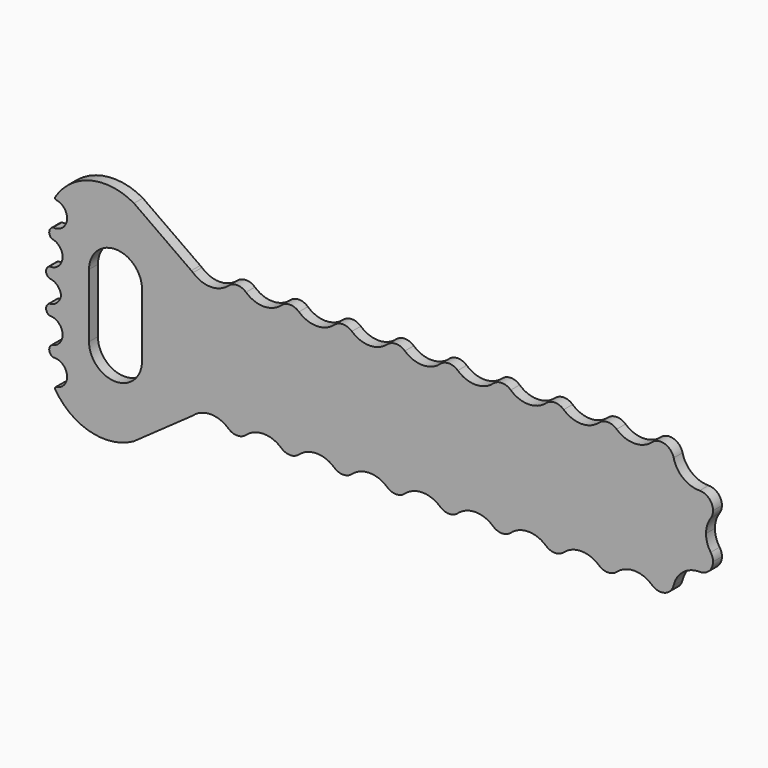
from build123d import *

# Parameters (mm, degrees)
F0_TEXT_SIZE = 24.3191204023
F1_DEPTH     = 2.667


# Not quite as in the source:
# - Text() gives the source's letters only with a copy of the font that has no kerning and outlines rounded to 1/6400 em; it was checked with that copy


with BuildPart() as f1:
    # F0 (on Front) → F1 (new body)
    with BuildSketch(Plane.XZ):
        with BuildLine():
            ThreePointArc((-63.1726785847, 1.1586809485), (-62.3909800512, 0.0883639945), (-62.1143452513, -1.2078243277))
            ThreePointArc((-62.1143452513, -1.2078243277), (-68.0745680167, -2.732015637), (-63.5777525882, 1.4663251737))
            Line((-63.5777525882, 1.4663251737), (-77.3401691147, 11.2148536242))
            ThreePointArc((-77.3401691147, 11.2148536242), (-87.8068892458, 12.6196854607), (-96.2739288474, 6.3081861795))
            ThreePointArc((-96.2739288474, 6.3081861795), (-96.2289020352, 6.0064040212), (-95.9839214808, 5.8245128095))
            ThreePointArc((-95.9839214808, 5.8245128095), (-93.4015593805, 2.4408889862), (-96.7397936857, -0.199886642))
            ThreePointArc((-96.7397936857, -0.199886642), (-97.6524269014, -1.3446739458), (-97.0623695413, -2.6845506823))
            ThreePointArc((-97.0623695413, -2.6845506823), (-94.4816228819, -5.9852371965), (-97.6549069574, -8.7211196796))
            ThreePointArc((-97.6549069574, -8.7211196796), (-98.4182841729, -9.9748064549), (-97.6549069574, -11.2284932301))
            ThreePointArc((-97.6549069574, -11.2284932301), (-95.7570755771, -12.0560699309), (-94.8309801189, -13.9078243277))
            ThreePointArc((-94.8309801189, -13.9078243277), (-95.7570755771, -15.7595787244), (-97.6549069574, -16.5871554253))
            ThreePointArc((-97.6549069574, -16.5871554253), (-98.4182841729, -17.8408422005), (-97.6549069574, -19.0945289757))
            ThreePointArc((-97.6549069574, -19.0945289757), (-94.4816228819, -21.8304114589), (-97.0623695413, -25.131097973))
            ThreePointArc((-97.0623695413, -25.131097973), (-97.6524269014, -26.4709747096), (-96.7397936857, -27.6157620133))
            ThreePointArc((-96.7397936857, -27.6157620133), (-93.4015593805, -30.2565376416), (-95.9839214808, -33.6401614649))
            ThreePointArc((-95.9839214808, -33.6401614649), (-96.2289020352, -33.8220526766), (-96.2739288474, -34.1238348349))
            ThreePointArc((-96.2739288474, -34.1238348349), (-87.8068892458, -40.4353341161), (-77.3401691147, -39.0305022795))
            Line((-77.3401691147, -39.0305022795), (-63.5777525882, -29.281973829))
            ThreePointArc((-63.5777525882, -29.281973829), (-68.0745680167, -25.0836330184), (-62.1143452513, -26.6078243277))
            ThreePointArc((-62.1143452513, -26.6078243277), (-62.3909800512, -27.9040126499), (-63.1726785847, -28.9743296039))
            ThreePointArc((-63.1726785847, -28.9743296039), (-58.9393452513, -27.3573401562), (-54.706011918, -28.9743296039))
            ThreePointArc((-54.706011918, -28.9743296039), (-53.8855335735, -23.7094591276), (-49.4143452513, -26.6078243277))
            ThreePointArc((-49.4143452513, -26.6078243277), (-49.6909800512, -27.9040126499), (-50.4726785847, -28.9743296039))
            ThreePointArc((-50.4726785847, -28.9743296039), (-46.2393452513, -27.3573401562), (-42.006011918, -28.9743296039))
            ThreePointArc((-42.006011918, -28.9743296039), (-41.1855335735, -23.7094591276), (-36.7143452513, -26.6078243277))
            ThreePointArc((-36.7143452513, -26.6078243277), (-36.9909800512, -27.9040126499), (-37.7726785847, -28.9743296039))
            ThreePointArc((-37.7726785847, -28.9743296039), (-33.5393452513, -27.3573401562), (-29.306011918, -28.9743296039))
            ThreePointArc((-29.306011918, -28.9743296039), (-28.4855335735, -23.7094591276), (-24.0143452513, -26.6078243277))
            ThreePointArc((-24.0143452513, -26.6078243277), (-24.2909800512, -27.9040126499), (-25.0726785847, -28.9743296039))
            ThreePointArc((-25.0726785847, -28.9743296039), (-20.8393452513, -27.3573401562), (-16.606011918, -28.9743296039))
            ThreePointArc((-16.606011918, -28.9743296039), (-15.7855335735, -23.7094591276), (-11.3143452513, -26.6078243277))
            ThreePointArc((-11.3143452513, -26.6078243277), (-11.5909800512, -27.9040126499), (-12.3726785847, -28.9743296039))
            ThreePointArc((-12.3726785847, -28.9743296039), (-8.1393452513, -27.3573401562), (-3.906011918, -28.9743296039))
            ThreePointArc((-3.906011918, -28.9743296039), (-3.0855335735, -23.7094591276), (1.3856547487, -26.6078243277))
            ThreePointArc((1.3856547487, -26.6078243277), (1.1090199488, -27.9040126499), (0.3273214153, -28.9743296039))
            ThreePointArc((0.3273214153, -28.9743296039), (4.5606547487, -27.3573401562), (8.793988082, -28.9743296039))
            ThreePointArc((8.793988082, -28.9743296039), (9.6144664265, -23.7094591276), (14.0856547487, -26.6078243277))
            ThreePointArc((14.0856547487, -26.6078243277), (13.8090199488, -27.9040126499), (13.0273214153, -28.9743296039))
            ThreePointArc((13.0273214153, -28.9743296039), (17.2606547487, -27.3573401562), (21.493988082, -28.9743296039))
            ThreePointArc((21.493988082, -28.9743296039), (22.3144664265, -23.7094591276), (26.7856547487, -26.6078243277))
            ThreePointArc((26.7856547487, -26.6078243277), (26.5090199488, -27.9040126499), (25.7273214153, -28.9743296039))
            ThreePointArc((25.7273214153, -28.9743296039), (29.9606547487, -27.3573401562), (34.193988082, -28.9743296039))
            ThreePointArc((34.193988082, -28.9743296039), (35.0144664265, -23.7094591276), (39.4856547487, -26.6078243277))
            ThreePointArc((39.4856547487, -26.6078243277), (39.2090199488, -27.9040126499), (38.4273214153, -28.9743296039))
            ThreePointArc((38.4273214153, -28.9743296039), (42.6606547487, -27.3573401562), (46.893988082, -28.9743296039))
            ThreePointArc((46.893988082, -28.9743296039), (47.7144664265, -23.7094591276), (52.1856547487, -26.6078243277))
            ThreePointArc((52.1856547487, -26.6078243277), (52.1636501137, -26.9809800972), (52.097941219, -27.3489634846))
            ThreePointArc((52.097941219, -27.3489634846), (54.3639551489, -23.8266772361), (58.3302922873, -22.4815046631))
            ThreePointArc((58.3302922873, -22.4815046631), (55.5557401714, -17.8162191901), (60.9749127444, -17.5070321728))
            ThreePointArc((60.9749127444, -17.5070321728), (60.1424539989, -15.7923284143), (59.856375531, -13.9078243277))
            ThreePointArc((59.856375531, -13.9078243277), (60.1424539989, -12.023320241), (60.9749127444, -10.3086164825))
            ThreePointArc((60.9749127444, -10.3086164825), (55.5557401714, -9.9994294652), (58.3302922873, -5.3341439923))
            ThreePointArc((58.3302922873, -5.3341439923), (54.3639551489, -3.9889714193), (52.097941219, -0.4666851708))
            ThreePointArc((52.097941219, -0.4666851708), (52.1636501137, -0.8346685582), (52.1856547487, -1.2078243277))
            ThreePointArc((52.1856547487, -1.2078243277), (47.7144664265, -4.1061895278), (46.893988082, 1.1586809485))
            ThreePointArc((46.893988082, 1.1586809485), (42.6606547487, -0.4583084991), (38.4273214153, 1.1586809485))
            ThreePointArc((38.4273214153, 1.1586809485), (39.2090199488, 0.0883639945), (39.4856547487, -1.2078243277))
            ThreePointArc((39.4856547487, -1.2078243277), (35.0144664265, -4.1061895278), (34.193988082, 1.1586809485))
            ThreePointArc((34.193988082, 1.1586809485), (29.9606547487, -0.4583084991), (25.7273214153, 1.1586809485))
            ThreePointArc((25.7273214153, 1.1586809485), (26.5090199488, 0.0883639945), (26.7856547487, -1.2078243277))
            ThreePointArc((26.7856547487, -1.2078243277), (22.3144664265, -4.1061895278), (21.493988082, 1.1586809485))
            ThreePointArc((21.493988082, 1.1586809485), (17.2606547487, -0.4583084991), (13.0273214153, 1.1586809485))
            ThreePointArc((13.0273214153, 1.1586809485), (13.8090199488, 0.0883639945), (14.0856547487, -1.2078243277))
            ThreePointArc((14.0856547487, -1.2078243277), (9.6144664265, -4.1061895278), (8.793988082, 1.1586809485))
            ThreePointArc((8.793988082, 1.1586809485), (4.5606547487, -0.4583084991), (0.3273214153, 1.1586809485))
            ThreePointArc((0.3273214153, 1.1586809485), (1.1090199488, 0.0883639945), (1.3856547487, -1.2078243277))
            ThreePointArc((1.3856547487, -1.2078243277), (-3.0855335735, -4.1061895278), (-3.906011918, 1.1586809485))
            ThreePointArc((-3.906011918, 1.1586809485), (-8.1393452513, -0.4583084991), (-12.3726785847, 1.1586809485))
            ThreePointArc((-12.3726785847, 1.1586809485), (-11.5909800512, 0.0883639945), (-11.3143452513, -1.2078243277))
            ThreePointArc((-11.3143452513, -1.2078243277), (-15.7855335735, -4.1061895278), (-16.606011918, 1.1586809485))
            ThreePointArc((-16.606011918, 1.1586809485), (-20.8393452513, -0.4583084991), (-25.0726785847, 1.1586809485))
            ThreePointArc((-25.0726785847, 1.1586809485), (-24.2909800512, 0.0883639945), (-24.0143452513, -1.2078243277))
            ThreePointArc((-24.0143452513, -1.2078243277), (-28.4855335735, -4.1061895278), (-29.306011918, 1.1586809485))
            ThreePointArc((-29.306011918, 1.1586809485), (-33.5393452513, -0.4583084991), (-37.7726785847, 1.1586809485))
            ThreePointArc((-37.7726785847, 1.1586809485), (-36.9909800512, 0.0883639945), (-36.7143452513, -1.2078243277))
            ThreePointArc((-36.7143452513, -1.2078243277), (-41.1855335735, -4.1061895278), (-42.006011918, 1.1586809485))
            ThreePointArc((-42.006011918, 1.1586809485), (-46.2393452513, -0.4583084991), (-50.4726785847, 1.1586809485))
            ThreePointArc((-50.4726785847, 1.1586809485), (-49.6909800512, 0.0883639945), (-49.4143452513, -1.2078243277))
            ThreePointArc((-49.4143452513, -1.2078243277), (-53.8855335735, -4.1061895278), (-54.706011918, 1.1586809485))
            ThreePointArc((-54.706011918, 1.1586809485), (-58.9393452513, -0.4583084991), (-63.1726785847, 1.1586809485))
        make_face()
        with BuildLine():
            Line((-75.4171005012, -6.2992), (-75.4171005012, -13.9078243277))
            Line((-75.4171005012, -13.9078243277), (-75.4171005012, -21.5164486554))
            ThreePointArc((-75.4171005012, -21.5164486554), (-75.4170897429, -21.5281375467), (-75.4171005012, -21.539826438))
            ThreePointArc((-75.4171005012, -21.539826438), (-81.7671005012, -27.8781483049), (-88.1171005012, -21.539826438))
            Line((-88.1171005012, -21.539826438), (-88.1171005012, -21.5164486554))
            Line((-88.1171005012, -21.5164486554), (-88.1171005012, -13.9078243277))
            Line((-88.1171005012, -13.9078243277), (-88.1171005012, -6.2992))
            Line((-88.1171005012, -6.2992), (-88.1171005012, -6.2758222174))
            ThreePointArc((-88.1171005012, -6.2758222174), (-81.7671005012, 0.0624996496), (-75.4171005012, -6.2758222174))
            Line((-75.4171005012, -6.2758222174), (-75.4171005012, -6.2992))
        make_face(mode=Mode.SUBTRACT)
        with BuildLine():
            add(Edge.make_bspline(
                [(-19.9713112204, -7.2212566106), (-17.8699872231, -9.5961707124), (-17.8699872231, -13.7760195316)],
                knots=[0, 0, 0, 1, 1, 1], degree=2))
            add(Edge.make_bspline(
                [(-17.8699872231, -13.7760195316), (-17.8699872231, -17.944468763), (-19.9789109455, -20.3326823838)],
                knots=[0, 0, 0, 1, 1, 1], degree=2))
            add(Edge.make_bspline(
                [(-19.9789109455, -20.3326823838), (-22.0878346679, -22.7208960045), (-25.8382990175, -22.7208960045)],
                knots=[0, 0, 0, 1, 1, 1], degree=2))
            add(Edge.make_bspline(
                [(-25.8382990175, -22.7208960045), (-29.6723603434, -22.7208960045), (-31.7565849591, -20.374480872)],
                knots=[0, 0, 0, 1, 1, 1], degree=2))
            add(Edge.make_bspline(
                [(-31.7565849591, -20.374480872), (-33.8408095749, -18.0280657394), (-33.8408095749, -13.7532203562)],
                knots=[0, 0, 0, 1, 1, 1], degree=2))
            add(Edge.make_bspline(
                [(-33.8408095749, -13.7532203562), (-33.8408095749, -9.512573736), (-31.7508851653, -7.1794581224)],
                knots=[0, 0, 0, 1, 1, 1], degree=2))
            add(Edge.make_bspline(
                [(-31.7508851653, -7.1794581224), (-29.6609607557, -4.8463425088), (-25.8154998421, -4.8463425088)],
                knots=[0, 0, 0, 1, 1, 1], degree=2))
            add(Edge.make_bspline(
                [(-25.8154998421, -4.8463425088), (-22.0726352177, -4.8463425088), (-19.9713112204, -7.2212566106)],
                knots=[0, 0, 0, 1, 1, 1], degree=2))
        make_face(mode=Mode.SUBTRACT)
        Polygon((-8.6591203708, -6.913467743), (-8.6591203708, -22.4815046631), (-10.6768473916, -22.4815046631), (-10.6768473916, -6.913467743), (-16.1752485201, -6.913467743), (-16.1752485201, -5.1199326133), (-3.1607192423, -5.1199326133), (-3.1607192423, -6.913467743), align=None, mode=Mode.SUBTRACT)
        Polygon((12.6353094316, -5.1199326133), (12.6353094316, -22.4815046631), (10.6175824107, -22.4815046631), (10.6175824107, -14.3118001529), (1.4713132219, -14.3118001529), (1.4713132219, -22.4815046631), (-0.546413799, -22.4815046631), (-0.546413799, -5.1199326133), (1.4713132219, -5.1199326133), (1.4713132219, -12.5068654356), (10.6175824107, -12.5068654356), (10.6175824107, -5.1199326133), align=None, mode=Mode.SUBTRACT)
        with BuildLine():
            Line((25.0342609742, -15.1895684049), (25.0342609742, -13.3846336876))
            Line((25.0342609742, -13.3846336876), (30.9354475343, -13.3846336876))
            Line((30.9354475343, -13.3846336876), (30.9354475343, -21.8279283023))
            add(Edge.make_bspline(
                [(30.9354475343, -21.8279283023), (29.556097424, -22.2687123596), (28.1311489629, -22.494804182)],
                knots=[0, 0, 0, 1, 1, 1], degree=2))
            add(Edge.make_bspline(
                [(28.1311489629, -22.494804182), (26.7062005018, -22.7208960045), (24.8290683958, -22.7208960045)],
                knots=[0, 0, 0, 1, 1, 1], degree=2))
            add(Edge.make_bspline(
                [(24.8290683958, -22.7208960045), (20.8886109181, -22.7208960045), (18.6922903568, -20.374480872)],
                knots=[0, 0, 0, 1, 1, 1], degree=2))
            add(Edge.make_bspline(
                [(18.6922903568, -20.374480872), (16.4959697954, -18.0280657394), (16.4959697954, -13.8026185695)],
                knots=[0, 0, 0, 1, 1, 1], degree=2))
            add(Edge.make_bspline(
                [(16.4959697954, -13.8026185695), (16.4959697954, -11.0933165622), (17.5827304884, -9.0565902285)],
                knots=[0, 0, 0, 1, 1, 1], degree=2))
            add(Edge.make_bspline(
                [(17.5827304884, -9.0565902285), (18.6694911814, -7.0198638948), (20.7119173089, -5.9464027208)],
                knots=[0, 0, 0, 1, 1, 1], degree=2))
            add(Edge.make_bspline(
                [(20.7119173089, -5.9464027208), (22.7543434365, -4.8729415468), (25.4940443443, -4.8729415468)],
                knots=[0, 0, 0, 1, 1, 1], degree=2))
            add(Edge.make_bspline(
                [(25.4940443443, -4.8729415468), (28.2755437403, -4.8729415468), (30.6732570175, -5.8913047136)],
                knots=[0, 0, 0, 1, 1, 1], degree=2))
            Line((30.6732570175, -5.8913047136), (29.8904853295, -7.6734402556))
            add(Edge.make_bspline(
                [(29.8904853295, -7.6734402556), (27.5383704031, -6.6778762641), (25.3648490172, -6.6778762641)],
                knots=[0, 0, 0, 1, 1, 1], degree=2))
            add(Edge.make_bspline(
                [(25.3648490172, -6.6778762641), (22.1957636397, -6.6778762641), (20.4136280977, -8.5645080266)],
                knots=[0, 0, 0, 1, 1, 1], degree=2))
            add(Edge.make_bspline(
                [(20.4136280977, -8.5645080266), (18.6314925558, -10.451139789), (18.6314925558, -13.8026185695)],
                knots=[0, 0, 0, 1, 1, 1], degree=2))
            add(Edge.make_bspline(
                [(18.6314925558, -13.8026185695), (18.6314925558, -17.3174914401), (20.3471305029, -19.1338257452)],
                knots=[0, 0, 0, 1, 1, 1], degree=2))
            add(Edge.make_bspline(
                [(20.3471305029, -19.1338257452), (22.06276845, -20.9501600502), (25.3876481925, -20.9501600502)],
                knots=[0, 0, 0, 1, 1, 1], degree=2))
            add(Edge.make_bspline(
                [(25.3876481925, -20.9501600502), (27.1925829099, -20.9501600502), (28.9139206509, -20.5321751683)],
                knots=[0, 0, 0, 1, 1, 1], degree=2))
            Line((28.9139206509, -20.5321751683), (28.9139206509, -15.1895684049))
            Line((28.9139206509, -15.1895684049), (25.0342609742, -15.1895684049))
        make_face(mode=Mode.SUBTRACT)
        with BuildLine():
            ThreePointArc((-63.5777525882, 1.4663251737), (-68.0745680167, -2.732015637), (-62.1143452513, -1.2078243277))
            ThreePointArc((-62.1143452513, -1.2078243277), (-62.3909800512, 0.0883639945), (-63.1726785847, 1.1586809485))
            ThreePointArc((-63.1726785847, 1.1586809485), (-63.3690448539, 1.3206280416), (-63.5777525882, 1.4663251737))
        make_face()
        with BuildLine():
            ThreePointArc((-50.4726785847, 1.1586809485), (-52.5893452513, 1.9671756723), (-54.706011918, 1.1586809485))
            ThreePointArc((-54.706011918, 1.1586809485), (-53.8855335735, -4.1061895278), (-49.4143452513, -1.2078243277))
            ThreePointArc((-49.4143452513, -1.2078243277), (-49.6909800512, 0.0883639945), (-50.4726785847, 1.1586809485))
        make_face()
        with BuildLine():
            ThreePointArc((-37.7726785847, 1.1586809485), (-39.8893452513, 1.9671756723), (-42.006011918, 1.1586809485))
            ThreePointArc((-42.006011918, 1.1586809485), (-41.1855335735, -4.1061895278), (-36.7143452513, -1.2078243277))
            ThreePointArc((-36.7143452513, -1.2078243277), (-36.9909800512, 0.0883639945), (-37.7726785847, 1.1586809485))
        make_face()
        with BuildLine():
            ThreePointArc((-25.0726785847, 1.1586809485), (-27.1893452513, 1.9671756723), (-29.306011918, 1.1586809485))
            ThreePointArc((-29.306011918, 1.1586809485), (-28.4855335735, -4.1061895278), (-24.0143452513, -1.2078243277))
            ThreePointArc((-24.0143452513, -1.2078243277), (-24.2909800512, 0.0883639945), (-25.0726785847, 1.1586809485))
        make_face()
        with BuildLine():
            ThreePointArc((-12.3726785847, 1.1586809485), (-14.4893452513, 1.9671756723), (-16.606011918, 1.1586809485))
            ThreePointArc((-16.606011918, 1.1586809485), (-15.7855335735, -4.1061895278), (-11.3143452513, -1.2078243277))
            ThreePointArc((-11.3143452513, -1.2078243277), (-11.5909800512, 0.0883639945), (-12.3726785847, 1.1586809485))
        make_face()
        with BuildLine():
            ThreePointArc((0.3273214153, 1.1586809485), (-1.7893452513, 1.9671756723), (-3.906011918, 1.1586809485))
            ThreePointArc((-3.906011918, 1.1586809485), (-3.0855335735, -4.1061895278), (1.3856547487, -1.2078243277))
            ThreePointArc((1.3856547487, -1.2078243277), (1.1090199488, 0.0883639945), (0.3273214153, 1.1586809485))
        make_face()
        with BuildLine():
            ThreePointArc((13.0273214153, 1.1586809485), (10.9106547487, 1.9671756723), (8.793988082, 1.1586809485))
            ThreePointArc((8.793988082, 1.1586809485), (9.6144664265, -4.1061895278), (14.0856547487, -1.2078243277))
            ThreePointArc((14.0856547487, -1.2078243277), (13.8090199488, 0.0883639945), (13.0273214153, 1.1586809485))
        make_face()
        with BuildLine():
            ThreePointArc((25.7273214153, 1.1586809485), (23.6106547487, 1.9671756723), (21.493988082, 1.1586809485))
            ThreePointArc((21.493988082, 1.1586809485), (22.3144664265, -4.1061895278), (26.7856547487, -1.2078243277))
            ThreePointArc((26.7856547487, -1.2078243277), (26.5090199488, 0.0883639945), (25.7273214153, 1.1586809485))
        make_face()
        with BuildLine():
            ThreePointArc((38.4273214153, 1.1586809485), (36.3106547487, 1.9671756723), (34.193988082, 1.1586809485))
            ThreePointArc((34.193988082, 1.1586809485), (35.0144664265, -4.1061895278), (39.4856547487, -1.2078243277))
            ThreePointArc((39.4856547487, -1.2078243277), (39.2090199488, 0.0883639945), (38.4273214153, 1.1586809485))
        make_face()
        with BuildLine():
            ThreePointArc((52.097941219, -0.4666851708), (49.9572166623, 1.8227936858), (46.893988082, 1.1586809485))
            ThreePointArc((46.893988082, 1.1586809485), (47.7144664265, -4.1061895278), (52.1856547487, -1.2078243277))
            ThreePointArc((52.1856547487, -1.2078243277), (52.1636501137, -0.8346685582), (52.097941219, -0.4666851708))
        make_face()
        with BuildLine():
            ThreePointArc((61.5341813511, -8.50901256), (60.5940082149, -6.2537578318), (58.3302922873, -5.3341439923))
            ThreePointArc((58.3302922873, -5.3341439923), (55.5557401714, -9.9994294652), (60.9749127444, -10.3086164825))
            ThreePointArc((60.9749127444, -10.3086164825), (61.3911421172, -9.4512646033), (61.5341813511, -8.50901256))
        make_face()
        with BuildLine():
            ThreePointArc((61.5341813511, -19.3066360954), (61.3911421172, -18.3643840521), (60.9749127444, -17.5070321728))
            ThreePointArc((60.9749127444, -17.5070321728), (55.5557401714, -17.8162191901), (58.3302922873, -22.4815046631))
            ThreePointArc((58.3302922873, -22.4815046631), (60.5940082149, -21.5618908235), (61.5341813511, -19.3066360954))
        make_face()
        with BuildLine():
            ThreePointArc((46.893988082, -28.9743296039), (49.9572166623, -29.6384423412), (52.097941219, -27.3489634846))
            ThreePointArc((52.097941219, -27.3489634846), (52.1636501137, -26.9809800972), (52.1856547487, -26.6078243277))
            ThreePointArc((52.1856547487, -26.6078243277), (47.7144664265, -23.7094591276), (46.893988082, -28.9743296039))
        make_face()
        with BuildLine():
            ThreePointArc((34.193988082, -28.9743296039), (36.3106547487, -29.7828243277), (38.4273214153, -28.9743296039))
            ThreePointArc((38.4273214153, -28.9743296039), (39.2090199488, -27.9040126499), (39.4856547487, -26.6078243277))
            ThreePointArc((39.4856547487, -26.6078243277), (35.0144664265, -23.7094591276), (34.193988082, -28.9743296039))
        make_face()
        with BuildLine():
            ThreePointArc((21.493988082, -28.9743296039), (23.6106547487, -29.7828243277), (25.7273214153, -28.9743296039))
            ThreePointArc((25.7273214153, -28.9743296039), (26.5090199488, -27.9040126499), (26.7856547487, -26.6078243277))
            ThreePointArc((26.7856547487, -26.6078243277), (22.3144664265, -23.7094591276), (21.493988082, -28.9743296039))
        make_face()
        with BuildLine():
            ThreePointArc((14.0856547487, -26.6078243277), (9.6144664265, -23.7094591276), (8.793988082, -28.9743296039))
            ThreePointArc((8.793988082, -28.9743296039), (10.9106547487, -29.7828243277), (13.0273214153, -28.9743296039))
            ThreePointArc((13.0273214153, -28.9743296039), (13.8090199488, -27.9040126499), (14.0856547487, -26.6078243277))
        make_face()
        with BuildLine():
            ThreePointArc((1.3856547487, -26.6078243277), (-3.0855335735, -23.7094591276), (-3.906011918, -28.9743296039))
            ThreePointArc((-3.906011918, -28.9743296039), (-1.7893452513, -29.7828243277), (0.3273214153, -28.9743296039))
            ThreePointArc((0.3273214153, -28.9743296039), (1.1090199488, -27.9040126499), (1.3856547487, -26.6078243277))
        make_face()
        with BuildLine():
            ThreePointArc((-11.3143452513, -26.6078243277), (-15.7855335735, -23.7094591276), (-16.606011918, -28.9743296039))
            ThreePointArc((-16.606011918, -28.9743296039), (-14.4893452513, -29.7828243277), (-12.3726785847, -28.9743296039))
            ThreePointArc((-12.3726785847, -28.9743296039), (-11.5909800512, -27.9040126499), (-11.3143452513, -26.6078243277))
        make_face()
        with BuildLine():
            ThreePointArc((-24.0143452513, -26.6078243277), (-28.4855335735, -23.7094591276), (-29.306011918, -28.9743296039))
            ThreePointArc((-29.306011918, -28.9743296039), (-27.1893452513, -29.7828243277), (-25.0726785847, -28.9743296039))
            ThreePointArc((-25.0726785847, -28.9743296039), (-24.2909800512, -27.9040126499), (-24.0143452513, -26.6078243277))
        make_face()
        with BuildLine():
            ThreePointArc((-36.7143452513, -26.6078243277), (-41.1855335735, -23.7094591276), (-42.006011918, -28.9743296039))
            ThreePointArc((-42.006011918, -28.9743296039), (-39.8893452513, -29.7828243277), (-37.7726785847, -28.9743296039))
            ThreePointArc((-37.7726785847, -28.9743296039), (-36.9909800512, -27.9040126499), (-36.7143452513, -26.6078243277))
        make_face()
        with BuildLine():
            ThreePointArc((-49.4143452513, -26.6078243277), (-53.8855335735, -23.7094591276), (-54.706011918, -28.9743296039))
            ThreePointArc((-54.706011918, -28.9743296039), (-52.5893452513, -29.7828243277), (-50.4726785847, -28.9743296039))
            ThreePointArc((-50.4726785847, -28.9743296039), (-49.6909800512, -27.9040126499), (-49.4143452513, -26.6078243277))
        make_face()
        with BuildLine():
            ThreePointArc((-62.1143452513, -26.6078243277), (-68.0745680167, -25.0836330184), (-63.5777525882, -29.281973829))
            ThreePointArc((-63.5777525882, -29.281973829), (-63.3690448539, -29.136276697), (-63.1726785847, -28.9743296039))
            ThreePointArc((-63.1726785847, -28.9743296039), (-62.3909800512, -27.9040126499), (-62.1143452513, -26.6078243277))
        make_face()
        with BuildLine():
            add(Edge.make_bspline(
                [(-30.2024411709, -8.4752112564), (-31.7052868145, -10.2991452865), (-31.7052868145, -13.7760195316)],
                knots=[0, 0, 0, 1, 1, 1], degree=2))
            add(Edge.make_bspline(
                [(-31.7052868145, -13.7760195316), (-31.7052868145, -17.3022919899), (-30.2024411709, -19.1262260201)],
                knots=[0, 0, 0, 1, 1, 1], degree=2))
            add(Edge.make_bspline(
                [(-30.2024411709, -19.1262260201), (-28.6995955273, -20.9501600502), (-25.8382990175, -20.9501600502)],
                knots=[0, 0, 0, 1, 1, 1], degree=2))
            add(Edge.make_bspline(
                [(-25.8382990175, -20.9501600502), (-22.9542033323, -20.9501600502), (-21.4817565891, -19.1338257452)],
                knots=[0, 0, 0, 1, 1, 1], degree=2))
            add(Edge.make_bspline(
                [(-21.4817565891, -19.1338257452), (-20.009309846, -17.3174914401), (-20.009309846, -13.7760195316)],
                knots=[0, 0, 0, 1, 1, 1], degree=2))
            add(Edge.make_bspline(
                [(-20.009309846, -13.7760195316), (-20.009309846, -10.2725462486), (-21.4760567953, -8.4619117374)],
                knots=[0, 0, 0, 1, 1, 1], degree=2))
            add(Edge.make_bspline(
                [(-21.4760567953, -8.4619117374), (-22.9428037446, -6.6512772262), (-25.8154998421, -6.6512772262)],
                knots=[0, 0, 0, 1, 1, 1], degree=2))
            add(Edge.make_bspline(
                [(-25.8154998421, -6.6512772262), (-28.6995955273, -6.6512772262), (-30.2024411709, -8.4752112564)],
                knots=[0, 0, 0, 1, 1, 1], degree=2))
        make_face()
        with Locations((-35.3265558369, -22.4815046631)):
            Text('OTHG', F0_TEXT_SIZE, font='Open Sans', text_align=(TextAlign.LEFT, TextAlign.BOTTOM))
    extrude(amount=F1_DEPTH)


solid = f1.part
